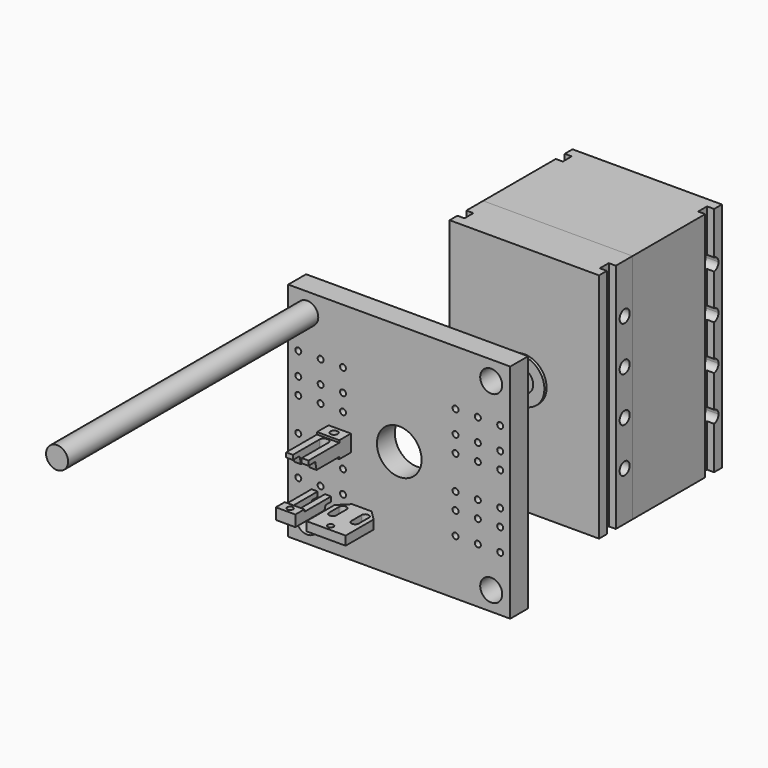
from build123d import *

# Parameters (mm, degrees)
F0_W      = 504.825
F0_H      = 504.825
F1_DEPTH  = 50.8
F2_R      = 25.019
F3_DEPTH  = 50.801
F5_D      = 13.49248
F5_DEPTH  = 38.1
F5_TIP    = 4.0535499425
F6_R      = 25.019
F7_DEPTH  = 711.2
F8_W      = 95.25
F8_H      = 527.05
F9_DEPTH  = 169.8625
F10_W     = 16.002
F10_H     = 25.4
F11_DEPTH = 527.051
F12_R     = 14.2875
F13_DEPTH = 29.21
F14_R     = 14.2875
F15_DEPTH = 25.4
F16_R     = 50.61585
F16_R_2   = 25.16505
F17_DEPTH = 6.35
F18_W     = 339.725
F18_H     = 527.05
F19_DEPTH = 254
F20_W     = 16.002
F20_H     = 25.4
F21_DEPTH = 527.051
F23_DEPTH = 29.21
F25_DEPTH = 29.21
F26_R     = 50.8
F27_DEPTH = 762.001
F28_W     = 101.6
F28_H     = 25.4
F29_DEPTH = 22.225
F31_D     = 13.49248
F32_W     = 16.51
F32_H     = 66.27876
F33_DEPTH = 276.226
F35_DEPTH = 274.6385
F36_W     = 76.2
F36_H     = 5.08
F37_DEPTH = 274.6385
F40_DEPTH = 88.9
F42_D     = 13.49248
F43_W     = 16.51
F43_H     = 50.8
F44_DEPTH = 271.146
F46_DEPTH = 20.32
F47_SIZE  = 22.225
F48_W     = 25.4
F48_H     = 5.08
F49_DEPTH = 388.9385
F51_DEPTH = 378.1435
F52_W     = 120.65
F52_H     = 37.9476
F53_DEPTH = 25.4
F55_DEPTH = 277.8135
F57_DEPTH = 376.7488423286
F59_D     = 16.66748
F60_W     = 87.63
F60_H     = 5.08
F61_DEPTH = 277.8135


# Not quite as in the source:
# - a pattern or mirror of a feature is missing from the dataset's text; its kind, count and spacing are read off the source's solid


with BuildPart() as f1:
    # F0 (on Front) → F1 (new body)
    with BuildSketch(Plane.XZ):
        Rectangle(F0_W, F0_H)
    extrude(amount=F1_DEPTH)

    # F2 (on face) → F3 (cut, through all)
    with BuildSketch(Plane.XZ.offset(50.8)):
        with Locations((-209.13725, 209.13725)):
            Circle(F2_R)
        with Locations((209.13725, 209.13725)):
            Circle(F2_R)
        with Locations((-209.13725, -209.13725)):
            Circle(F2_R)
        with Locations((209.13725, -209.13725)):
            Circle(F2_R)
    extrude(amount=-F3_DEPTH, mode=Mode.SUBTRACT)

    # F5
    with Locations(Plane.XZ.offset(50.8)):
        with Locations((-229.5525, 127), (-229.5525, 76.2), (-229.5525, 38.1), (-178.7525, 38.1), (-178.7525, 76.2), (-178.7525, 127), (-127.9525, 127), (-127.9525, 76.2), (-127.9525, 38.1), (-127.9525, -38.1), (-178.7525, -38.1), (-229.5525, -38.1), (-229.5525, -76.2), (-178.7525, -76.2), (-127.9525, -76.2), (-127.9525, -127), (-178.7525, -127), (-229.5525, -127), (127.9525, -127), (178.7525, -127), (229.5525, -127), (229.5525, -76.2), (178.7525, -76.2), (127.9525, -76.2), (127.9525, -38.1), (178.7525, -38.1), (229.5525, -38.1), (229.5525, 38.1), (178.7525, 38.1), (127.9525, 38.1), (127.9525, 76.2), (178.7525, 76.2), (229.5525, 76.2), (229.5525, 127), (178.7525, 127), (127.9525, 127)):
            Hole(F5_D / 2, depth=F5_DEPTH)
            with Locations((0, 0, -(F5_DEPTH + F5_TIP / 2))):  # 118° drill point
                Cone(0, F5_D / 2, F5_TIP, mode=Mode.SUBTRACT)

    # F26 (on face) → F27 (cut, through all)
    with BuildSketch(Plane(origin=(0, 0, 0), x_dir=(-1, 0, 0), z_dir=(0, 1, 0))):
        Circle(F26_R)
    extrude(amount=-F27_DEPTH, mode=Mode.SUBTRACT)


with BuildPart() as f7:
    # F6 (on face) → F7 (new body)
    with BuildSketch(Plane.XZ.offset(50.8)):
        with Locations((-209.13725, 209.13725)):
            Circle(F6_R)
    extrude(amount=F7_DEPTH)


with BuildPart() as f9:
    # F8 (on Right) → F9 (new body, symmetric)
    with BuildSketch(Plane.YZ):
        with Locations((352.425, 0)):
            Rectangle(F8_W, F8_H)
    extrude(amount=F9_DEPTH, both=True)

    # F10 (on face) → F11 (cut, through all)
    with BuildSketch(Plane.XY.offset(263.525)):
        with Locations((-161.8615, 339.725)):
            Rectangle(F10_W, F10_H)
        with Locations((161.8615, 339.725)):
            Rectangle(F10_W, F10_H)
    extrude(amount=-F11_DEPTH, mode=Mode.SUBTRACT)

    # F12 (on face) → F13 (cut)
    with BuildSketch(Plane.YZ.offset(169.8625)):
        with Locations((377.5837, 152.4)):
            Circle(F12_R)
        with Locations((377.5837, 50.8)):
            Circle(F12_R)
        with Locations((377.5837, -50.8)):
            Circle(F12_R)
        with Locations((377.5837, -152.4)):
            Circle(F12_R)
    extrude(amount=-F13_DEPTH, mode=Mode.SUBTRACT)

    # F14 (on face) → F15 (cut)
    with BuildSketch(Plane(origin=(-169.8625, 0, 0), x_dir=(0, -1, 0), z_dir=(-1, 0, 0))):
        with Locations((-377.5837, 152.4)):
            Circle(F14_R)
        with Locations((-377.5837, 50.8)):
            Circle(F14_R)
        with Locations((-377.5837, -50.8)):
            Circle(F14_R)
        with Locations((-377.5837, -152.4)):
            Circle(F14_R)
    extrude(amount=-F15_DEPTH, mode=Mode.SUBTRACT)

    # F16 (on face) → F17 (join)
    with BuildSketch(Plane.XZ.offset(-304.8)):
        Circle(F16_R)
        Circle(F16_R_2, mode=Mode.SUBTRACT)
    extrude(amount=F17_DEPTH)


with BuildPart() as f19:
    # F18 (on face) → F19 (new body)
    with BuildSketch(Plane(origin=(0, 400.05, 0), x_dir=(-1, 0, 0), z_dir=(0, 1, 0))):
        Rectangle(F18_W, F18_H)
    extrude(amount=F19_DEPTH)

    # F20 (on face) → F21 (cut, through all)
    with BuildSketch(Plane.XY.offset(263.525)):
        with Locations((-161.8615, 619.125)):
            Rectangle(F20_W, F20_H)
        with Locations((161.8615, 619.125)):
            Rectangle(F20_W, F20_H)
    extrude(amount=-F21_DEPTH, mode=Mode.SUBTRACT)

    # F22 (on face) → F23 (cut)
    with BuildSketch(Plane.YZ.offset(169.8625)):
        with BuildLine():
            ThreePointArc((631.825, 138.2172838846), (640.7938279134, 142.9275323635), (644.3853, 152.4))
            ThreePointArc((644.3853, 152.4), (640.7938279134, 161.8724676365), (631.825, 166.5827161154))
            Line((631.825, 166.5827161154), (631.825, 138.2172838846))
        make_face()
        with BuildLine():
            Line((631.825, 138.2172838846), (631.825, 166.5827161154))
            ThreePointArc((631.825, 166.5827161154), (615.8103, 152.4), (631.825, 138.2172838846))
        make_face()
        with BuildLine():
            Line((631.825, 36.6172838846), (631.825, 64.9827161154))
            ThreePointArc((631.825, 64.9827161154), (615.8103, 50.8), (631.825, 36.6172838846))
        make_face()
        with BuildLine():
            ThreePointArc((644.3853, 50.8), (640.7938279134, 60.2724676365), (631.825, 64.9827161154))
            Line((631.825, 64.9827161154), (631.825, 36.6172838846))
            ThreePointArc((631.825, 36.6172838846), (640.7938279134, 41.3275323635), (644.3853, 50.8))
        make_face()
        with BuildLine():
            Line((631.825, -64.9827161154), (631.825, -36.6172838846))
            ThreePointArc((631.825, -36.6172838846), (615.8103, -50.8), (631.825, -64.9827161154))
        make_face()
        with BuildLine():
            ThreePointArc((644.3853, -50.8), (640.7938279134, -41.3275323635), (631.825, -36.6172838846))
            Line((631.825, -36.6172838846), (631.825, -64.9827161154))
            ThreePointArc((631.825, -64.9827161154), (640.7938279134, -60.2724676365), (644.3853, -50.8))
        make_face()
        with BuildLine():
            Line((631.825, -138.2172838846), (631.825, -166.5827161154))
            ThreePointArc((631.825, -166.5827161154), (640.7938279134, -161.8724676365), (644.3853, -152.4))
            ThreePointArc((644.3853, -152.4), (640.7938279134, -142.9275323635), (631.825, -138.2172838846))
        make_face()
        with BuildLine():
            ThreePointArc((631.825, -138.2172838846), (615.8103, -152.4), (631.825, -166.5827161154))
            Line((631.825, -166.5827161154), (631.825, -138.2172838846))
        make_face()
    extrude(amount=-F23_DEPTH, mode=Mode.SUBTRACT)

    # F24 (on face) → F25 (cut)
    with BuildSketch(Plane(origin=(-169.8625, 0, 0), x_dir=(0, -1, 0), z_dir=(-1, 0, 0))):
        with BuildLine():
            ThreePointArc((-631.825, 138.2172838846), (-620.6253323635, 141.7039720866), (-615.8103, 152.4))
            ThreePointArc((-615.8103, 152.4), (-620.6253323635, 163.0960279134), (-631.825, 166.5827161154))
            Line((-631.825, 166.5827161154), (-631.825, 138.2172838846))
        make_face()
        with BuildLine():
            Line((-631.825, 138.2172838846), (-631.825, 166.5827161154))
            ThreePointArc((-631.825, 166.5827161154), (-644.3853, 152.4), (-631.825, 138.2172838846))
        make_face()
        with BuildLine():
            Line((-631.825, 36.6172838846), (-631.825, 64.9827161154))
            ThreePointArc((-631.825, 64.9827161154), (-644.3853, 50.8), (-631.825, 36.6172838846))
        make_face()
        with BuildLine():
            ThreePointArc((-615.8103, 50.8), (-620.6253323635, 61.4960279134), (-631.825, 64.9827161154))
            Line((-631.825, 64.9827161154), (-631.825, 36.6172838846))
            ThreePointArc((-631.825, 36.6172838846), (-620.6253323635, 40.1039720866), (-615.8103, 50.8))
        make_face()
        with BuildLine():
            Line((-631.825, -64.9827161154), (-631.825, -36.6172838846))
            ThreePointArc((-631.825, -36.6172838846), (-644.3853, -50.8), (-631.825, -64.9827161154))
        make_face()
        with BuildLine():
            ThreePointArc((-615.8103, -50.8), (-620.6253323635, -40.1039720866), (-631.825, -36.6172838846))
            Line((-631.825, -36.6172838846), (-631.825, -64.9827161154))
            ThreePointArc((-631.825, -64.9827161154), (-620.6253323635, -61.4960279134), (-615.8103, -50.8))
        make_face()
        with BuildLine():
            Line((-631.825, -138.2172838846), (-631.825, -166.5827161154))
            ThreePointArc((-631.825, -166.5827161154), (-620.6253323635, -163.0960279134), (-615.8103, -152.4))
            ThreePointArc((-615.8103, -152.4), (-620.6253323635, -141.7039720866), (-631.825, -138.2172838846))
        make_face()
        with BuildLine():
            ThreePointArc((-631.825, -138.2172838846), (-644.3853, -152.4), (-631.825, -166.5827161154))
            Line((-631.825, -166.5827161154), (-631.825, -138.2172838846))
        make_face()
    extrude(amount=-F25_DEPTH, mode=Mode.SUBTRACT)


with BuildPart() as f29:
    # F28 (on Right) → F29 (new body, symmetric)
    with BuildSketch(Plane.YZ):
        with Locations((-323.0243325233, 0)):
            Rectangle(F28_W, F28_H)
    extrude(amount=F29_DEPTH, both=True)

    # F31 (through all)
    with Locations(Plane.XY.offset(12.7)):
        with Locations((0, -361.1243325233)):
            Hole(F31_D / 2)

    # F32 (on face) → F33 (cut, through all)
    with BuildSketch(Plane.XY.offset(12.7)):
        with Locations((0, -305.3637125233)):
            Rectangle(F32_W, F32_H)
        with BuildLine():
            Line((8.255, -338.5030925233), (-8.255, -338.5030925233))
            ThreePointArc((-8.255, -338.5030925233), (0, -346.7580925233), (8.255, -338.5030925233))
        make_face()
    extrude(amount=-F33_DEPTH, mode=Mode.SUBTRACT)

    # F34 (on face) → F35 (cut, through all)
    with BuildSketch(Plane.YZ.offset(22.225)):
        Polygon((-272.2243325233, -12.7), (-272.2243325233, -3.175), (-288.0993325233, -3.175), (-291.2743325233, -12.7), align=None)
    extrude(amount=-F35_DEPTH, mode=Mode.SUBTRACT)

    # F36 (on face) → F37 (cut, through all)
    with BuildSketch(Plane.YZ.offset(22.225)):
        with Locations((-310.3243325233, 10.16)):
            Rectangle(F36_W, F36_H)
    extrude(amount=-F37_DEPTH, mode=Mode.SUBTRACT)


with BuildPart() as f40:
    # F39 (on offset) → F40 (new body)
    with BuildSketch(Plane.YZ.offset(47.625)):
        Polygon((-272.2243325233, 7.62), (-348.4243325233, 7.62), (-348.4243325233, 12.7), (-373.8243325233, 12.7), (-373.8243325233, -12.7), (-291.2743325233, -12.7), (-288.0993325233, -3.175), (-272.2243325233, -3.175), align=None)
    extrude(amount=F40_DEPTH)

    # F42 (through all)
    with Locations(Plane.XY.offset(12.7)):
        with Locations((92.075, -361.1243325233)):
            Hole(F42_D / 2)

    # F43 (on face) → F44 (cut, through all)
    with BuildSketch(Plane.XY.offset(7.62)):
        with Locations((66.675, -297.6243325233)):
            Rectangle(F43_W, F43_H)
        with BuildLine():
            Line((74.93, -323.0243325233), (58.42, -323.0243325233))
            ThreePointArc((58.42, -323.0243325233), (66.675, -331.2793325233), (74.93, -323.0243325233))
        make_face()
        with BuildLine():
            Line((125.73, -323.0243325233), (109.22, -323.0243325233))
            ThreePointArc((109.22, -323.0243325233), (117.475, -331.2793325233), (125.73, -323.0243325233))
        make_face()
        with Locations((117.475, -297.6243325233)):
            Rectangle(F43_W, F43_H)
    extrude(amount=-F44_DEPTH, mode=Mode.SUBTRACT)

    # F45 (on face) → F46 (join, through all)
    with BuildSketch(Plane.XY.offset(7.62)):
        with BuildLine():
            Line((74.93, -272.2243325233), (58.42, -272.2243325233))
            Line((58.42, -272.2243325233), (58.42, -294.4493325233))
            ThreePointArc((58.42, -294.4493325233), (66.675, -286.1943325233), (74.93, -294.4493325233))
            Line((74.93, -294.4493325233), (74.93, -272.2243325233))
        make_face()
        with BuildLine():
            Line((125.73, -272.2243325233), (109.22, -272.2243325233))
            Line((109.22, -272.2243325233), (109.22, -294.4493325233))
            ThreePointArc((109.22, -294.4493325233), (117.475, -286.1943325233), (125.73, -294.4493325233))
            Line((125.73, -294.4493325233), (125.73, -272.2243325233))
        make_face()
    extrude(amount=-F46_DEPTH)

    # F47
    f47_edges = [f40.edges().sort_by_distance(p)[0] for p in [
        (136.525, -272.224333, 2.2225),
        (47.625, -272.224333, 2.2225),
    ]]
    chamfer(f47_edges, length=F47_SIZE)

    # F48 (on face) → F49 (cut, through all)
    with BuildSketch(Plane.YZ.offset(136.525)):
        with Locations((-361.1243325233, 10.16)):
            Rectangle(F48_W, F48_H)
    extrude(amount=-F49_DEPTH, mode=Mode.SUBTRACT)

    # F50 (on face) → F51 (cut, through all)
    with BuildSketch(Plane.YZ.offset(125.73)):
        Polygon((-272.2243325233, -3.175), (-288.0993325233, -3.175), (-291.2743325233, -12.7), (-272.2243325233, -12.7), align=None)
    f51 = extrude(amount=-F51_DEPTH, mode=Mode.SUBTRACT)

    # F51_copies: F51 across plane
    add(f51.mirror(Plane(origin=(92.075, 0, 0), x_dir=(0, 0, 1), z_dir=(1, 0, 0))), mode=Mode.SUBTRACT)


with BuildPart() as f53:
    # F52 (on Right) → F53 (new body, symmetric)
    with BuildSketch(Plane.YZ):
        with Locations((-280.1719936848, 94.2490423286)):
            Rectangle(F52_W, F52_H)
    extrude(amount=F53_DEPTH, both=True)

    # F54 (on face) → F55 (cut, through all)
    with BuildSketch(Plane.YZ.offset(25.4)):
        Polygon((-321.4469936848, 97.7288423286), (-340.4969936848, 97.7288423286), (-340.4969936848, 75.2752423286), (-252.8669936848, 75.2752423286), (-252.8669936848, 80.0377423286), (-317.6369936848, 80.0377423286), align=None)
    extrude(amount=-F55_DEPTH, mode=Mode.SUBTRACT)

    # F56 (on face) → F57 (cut, through all)
    with BuildSketch(Plane.XY.offset(113.2228423286)):
        with BuildLine():
            Line((10.0076, -340.4969936848), (10.0076, -265.0335936848))
            ThreePointArc((10.0076, -265.0335936848), (0, -275.0411936848), (-10.0076, -265.0335936848))
            Line((-10.0076, -265.0335936848), (-10.0076, -340.4969936848))
            Line((-10.0076, -340.4969936848), (10.0076, -340.4969936848))
        make_face()
        with BuildLine():
            ThreePointArc((-10.0076, -265.0335936848), (0, -275.0411936848), (10.0076, -265.0335936848))
            ThreePointArc((10.0076, -265.0335936848), (0, -255.0259936848), (-10.0076, -265.0335936848))
        make_face()
    extrude(amount=-F57_DEPTH, mode=Mode.SUBTRACT)

    # F59 (through all)
    with Locations(Plane.XY.offset(113.2228423286)):
        with Locations((0, -236.0648936848)):
            Hole(F59_D / 2)

    # F60 (on face) → F61 (cut, through all)
    with BuildSketch(Plane.YZ.offset(25.4)):
        with Locations((-296.6819936848, 110.6828423286)):
            Rectangle(F60_W, F60_H)
    extrude(amount=-F61_DEPTH, mode=Mode.SUBTRACT)


solid = Compound([f1.part, f7.part, f9.part, f19.part, f29.part, f40.part, f53.part])
